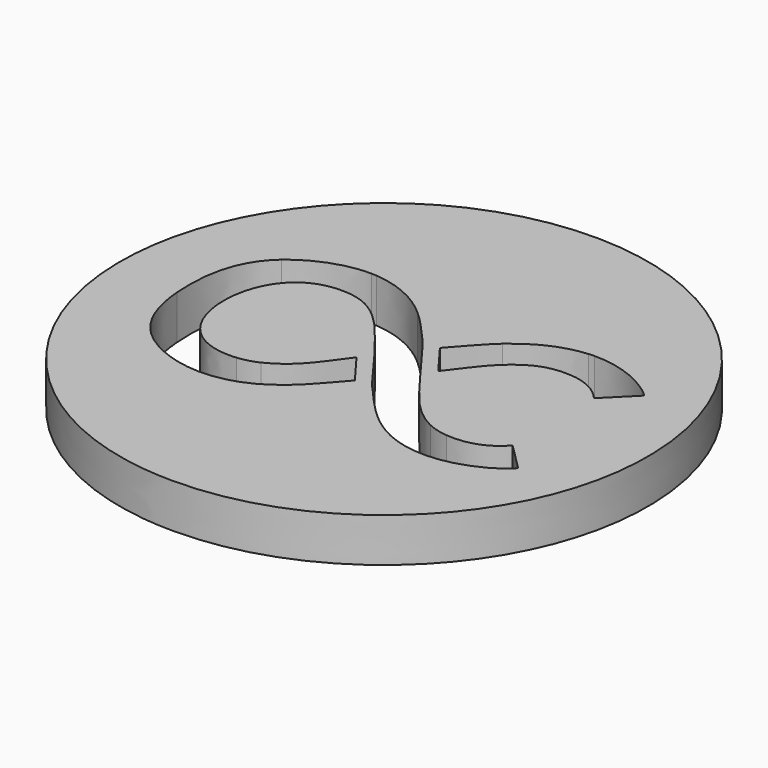
from build123d import *

# Parameters (mm, degrees)
F1_DEPTH = 2.5


# Not quite as in the source:
# - ends of sketch curves that miss each other by under 0.0002 mm in the source are joined


with BuildPart() as f1:
    # F0 (on Top) → F1 (new body)
    with BuildSketch(Plane.XY):
        with BuildLine():
            add(Edge.make_bspline(
                [(15, -0.0001027513), (15, 8.2842004769), (8.2843032282, 14.9996917461), (0, 14.9996917461)],
                knots=[0, 0, 0, 0, 1, 1, 1, 1], degree=3))
            add(Edge.make_bspline(
                [(0, 14.9996917461), (-8.2838816845, 14.9996917461), (-15, 8.2842004769), (-15, -0.0001027513)],
                knots=[0, 0, 0, 0, 1, 1, 1, 1], degree=3))
            add(Edge.make_bspline(
                [(-15, -0.0001027513), (-15, -8.2844049257), (-8.2838816845, -14.9996917461), (0, -14.9996917461)],
                knots=[0, 0, 0, 0, 1, 1, 1, 1], degree=3))
            add(Edge.make_bspline(
                [(0, -14.9996917461), (8.2843032282, -14.9996917461), (15, -8.2844049257), (15, -0.0001027513)],
                knots=[0, 0, 0, 0, 1, 1, 1, 1], degree=3))
        make_face()
        with BuildLine():
            add(Edge.make_bspline(
                [(-9.5178456332, 4.6235008323), (-8.5953951404, 5.4143422042), (-7.1139059696, 6.0933153489), (-5.5675201382, 6.0674114853)],
                knots=[0, 0, 0, 0, 1, 1, 1, 1], degree=3))
            add(Edge.make_bspline(
                [(-5.5675201382, 6.0674114853), (-5.4644547985, 6.0656821021), (-5.3610870012, 6.0607605787), (-5.2575642865, 6.052590007)],
                knots=[0, 0, 0, 0, 1, 1, 1, 1], degree=3))
            add(Edge.make_bspline(
                [(-5.2575642865, 6.052590007), (-3.7238869453, 5.932020063), (-2.5131816731, 5.1973346421), (-1.6472728438, 4.4363986379)],
                knots=[0, 0, 0, 0, 1, 1, 1, 1], degree=3))
            add(Edge.make_bspline(
                [(-1.6472728438, 4.4363986379), (-1.0359943564, 3.8993160663), (-0.4077814026, 3.1627263216), (0.2064489449, 2.4789370395)],
                knots=[0, 0, 0, 0, 1, 1, 1, 1], degree=3))
            add(Edge.make_bspline(
                [(0.2064489449, 2.4789370395), (0.2570373568, 2.422867505), (0.343813192, 2.3166711491), (0.4369806844, 2.2057977652)],
                knots=[0, 0, 0, 0, 1, 1, 1, 1], degree=3))
            Line((0.4369806844, 2.2057977652), (2.0786965277, -0.0048366876))
            add(Edge.make_bspline(
                [(2.0786965277, -0.0048366876), (2.0782749839, -0.0061013189), (2.0778534402, -0.0066704029), (2.0770525071, -0.0075134905)],
                knots=[0, 0, 0, 0, 1, 1, 1, 1], degree=3))
            add(Edge.make_bspline(
                [(2.0770525071, -0.0075134905), (3.1153832697, -1.3143855389), (4.0335529857, -2.9292764454), (5.5895742535, -3.6746153308)],
                knots=[0, 0, 0, 0, 1, 1, 1, 1], degree=3))
            add(Edge.make_bspline(
                [(5.5895742535, -3.6746153308), (5.9099685823, -3.8280667413), (6.3332332869, -3.9525486114), (6.7278245855, -3.985009588)],
                knots=[0, 0, 0, 0, 1, 1, 1, 1], degree=3))
            add(Edge.make_bspline(
                [(6.7278245855, -3.985009588), (8.0536671566, -4.0954614281), (9.0100276828, -3.6442578575), (9.643228553, -2.9128309698)],
                knots=[0, 0, 0, 0, 1, 1, 1, 1], degree=3))
            Line((9.643228553, -2.9128309698), (11.2028160809, -4.4734491721))
            add(Edge.make_bspline(
                [(11.2028160809, -4.4734491721), (10.8887459621, -4.7870977471), (10.5274007654, -5.0604330392), (10.1104665941, -5.2901901921)],
                knots=[0, 0, 0, 0, 1, 1, 1, 1], degree=3))
            add(Edge.make_bspline(
                [(10.1104665941, -5.2901901921), (9.301048843, -5.7366345338), (8.27868405, -6.0501366223), (7.2487852163, -6.0669994263)],
                knots=[0, 0, 0, 0, 1, 1, 1, 1], degree=3))
            add(Edge.make_bspline(
                [(7.2487852163, -6.0669994263), (4.4588242386, -6.1133724006), (2.893523739, -4.2754521794), (1.5562984327, -2.7421963821)],
                knots=[0, 0, 0, 0, 1, 1, 1, 1], degree=3))
            add(Edge.make_bspline(
                [(1.5562984327, -2.7421963821), (1.4441604176, -2.613195563), (1.3059320058, -2.4802533099), (1.1339316163, -2.2753693461)],
                knots=[0, 0, 0, 0, 1, 1, 1, 1], degree=3))
            add(Edge.make_bspline(
                [(1.1339316163, -2.2753693461), (1.0711173818, -2.2028596053), (0.9015419227, -1.9499597004), (0.8054236241, -1.8357129127)],
                knots=[0, 0, 0, 0, 1, 1, 1, 1], degree=3))
            Line((0.8054236241, -1.8357129127), (-0.5423645148, -0.0087443982))
            add(Edge.make_bspline(
                [(-0.5423645148, -0.0087443982), (-0.5423645148, -0.0083228545), (-0.5417321992, -0.0075113827), (-0.5413106554, -0.0075113827)],
                knots=[0, 0, 0, 0, 1, 1, 1, 1], degree=3))
            add(Edge.make_bspline(
                [(-0.5413106554, -0.0075113827), (-1.4460036177, 1.0797216167), (-2.4590596708, 2.6931887593), (-3.7284122175, 3.4735178838)],
                knots=[0, 0, 0, 0, 1, 1, 1, 1], degree=3))
            add(Edge.make_bspline(
                [(-3.7284122175, 3.4735178838), (-4.2941608181, 3.8213146643), (-4.961538348, 4.04057327), (-5.9079662495, 3.9710132816)],
                knots=[0, 0, 0, 0, 1, 1, 1, 1], degree=3))
            add(Edge.make_bspline(
                [(-5.9079662495, 3.9710132816), (-7.9407851168, 3.8213557648), (-8.9782222067, 2.0899554344), (-9.0629577702, 0.1789721962)],
                knots=[0, 0, 0, 0, 1, 1, 1, 1], degree=3))
            add(Edge.make_bspline(
                [(-9.0629577702, 0.1789721962), (-9.1573898938, -1.9727293862), (-7.9849945178, -4.2177154394), (-5.1920827339, -3.9850074803)],
                knots=[0, 0, 0, 0, 1, 1, 1, 1], degree=3))
            add(Edge.make_bspline(
                [(-5.1920827339, -3.9850074803), (-4.7974924891, -3.9525465037), (-4.3744227485, -3.8280646336), (-4.0544499634, -3.6746132231)],
                knots=[0, 0, 0, 0, 1, 1, 1, 1], degree=3))
            add(Edge.make_bspline(
                [(-4.0544499634, -3.6746132231), (-2.5924403294, -2.9743826808), (-2.0196150631, -1.8924326784), (-1.0546381827, -0.6336197793)],
                knots=[0, 0, 0, 0, 1, 1, 1, 1], degree=3))
            Line((-1.0546381827, -0.6336197793), (0.2661848562, -2.4029506166))
            add(Edge.make_bspline(
                [(0.2661848562, -2.4029506166), (0.1898801678, -2.507921334), (0.4391252883, -2.2315245804), (-0.4598473253, -3.2534867991)],
                knots=[0, 0, 0, 0, 1, 1, 1, 1], degree=3))
            add(Edge.make_bspline(
                [(-0.4598473253, -3.2534867991), (-1.358818885, -4.2754500717), (-2.924130977, -6.1133702929), (-5.7132488672, -6.0669973186)],
                knots=[0, 0, 0, 0, 1, 1, 1, 1], degree=3))
            add(Edge.make_bspline(
                [(-5.7132488672, -6.0669973186), (-6.7439918423, -6.0501345146), (-7.7655135478, -5.7366324261), (-8.574930245, -5.2901880844)],
                knots=[0, 0, 0, 0, 1, 1, 1, 1], degree=3))
            add(Edge.make_bspline(
                [(-8.574930245, -5.2901880844), (-10.1642555769, -4.4137406612), (-11.0010462716, -2.9361381239), (-11.1772631525, -0.7532412499)],
                knots=[0, 0, 0, 0, 1, 1, 1, 1], degree=3))
            add(Edge.make_bspline(
                [(-11.1772631525, -0.7532412499), (-11.3694997498, 1.6358052729), (-10.8597079208, 3.4730320546), (-9.5178456332, 4.6235008323)],
                knots=[0, 0, 0, 0, 1, 1, 1, 1], degree=3))
        make_face(mode=Mode.SUBTRACT)
        with BuildLine():
            add(Edge.make_bspline(
                [(6.7930700736, 6.052590007), (6.8965400953, 6.06073634), (6.9997982913, 6.0654945151), (7.1028478231, 6.067203875)],
                knots=[0, 0, 0, 0, 1, 1, 1, 1], degree=3))
            add(Edge.make_bspline(
                [(7.1028478231, 6.067203875), (8.6485876387, 6.0928474353), (10.1305320767, 5.4147321321), (11.0533798746, 4.623495563)],
                knots=[0, 0, 0, 0, 1, 1, 1, 1], degree=3))
            add(Edge.make_bspline(
                [(11.0533798746, 4.623495563), (11.109869899, 4.5745933262), (11.1634755102, 4.5236307943), (11.2170157822, 4.4726197848)],
                knots=[0, 0, 0, 0, 1, 1, 1, 1], degree=3))
            Line((11.2170157822, 4.4726197848), (9.6271698438, 2.8836021799))
            add(Edge.make_bspline(
                [(9.6271698438, 2.8836021799), (9.1090588488, 3.4910867735), (8.384025726, 3.9012477906), (7.443499437, 3.9708067251)],
                knots=[0, 0, 0, 0, 1, 1, 1, 1], degree=3))
            add(Edge.make_bspline(
                [(7.443499437, 3.9708067251), (6.4970715356, 4.0403667136), (5.8301060646, 3.8213136104), (5.2643564102, 3.4735168299)],
                knots=[0, 0, 0, 0, 1, 1, 1, 1], degree=3))
            add(Edge.make_bspline(
                [(5.2643564102, 3.4735168299), (4.0805846222, 2.7463053798), (3.4594957578, 1.6752080213), (2.6028619448, 0.6006213344)],
                knots=[0, 0, 0, 0, 1, 1, 1, 1], degree=3))
            Line((2.6028619448, 0.6006213344), (1.2682470482, 2.3876538477))
            add(Edge.make_bspline(
                [(1.2682470482, 2.3876538477), (1.9043945093, 3.0791415725), (2.4981525845, 3.8274418027), (3.1825731284, 4.4368096431)],
                knots=[0, 0, 0, 0, 1, 1, 1, 1], degree=3))
            add(Edge.make_bspline(
                [(3.1825731284, 4.4368096431), (4.0480593601, 5.1973251574), (5.2593927325, 5.932020063), (6.7930700736, 6.052590007)],
                knots=[0, 0, 0, 0, 1, 1, 1, 1], degree=3))
        make_face(mode=Mode.SUBTRACT)
    extrude(amount=F1_DEPTH)


solid = f1.part
